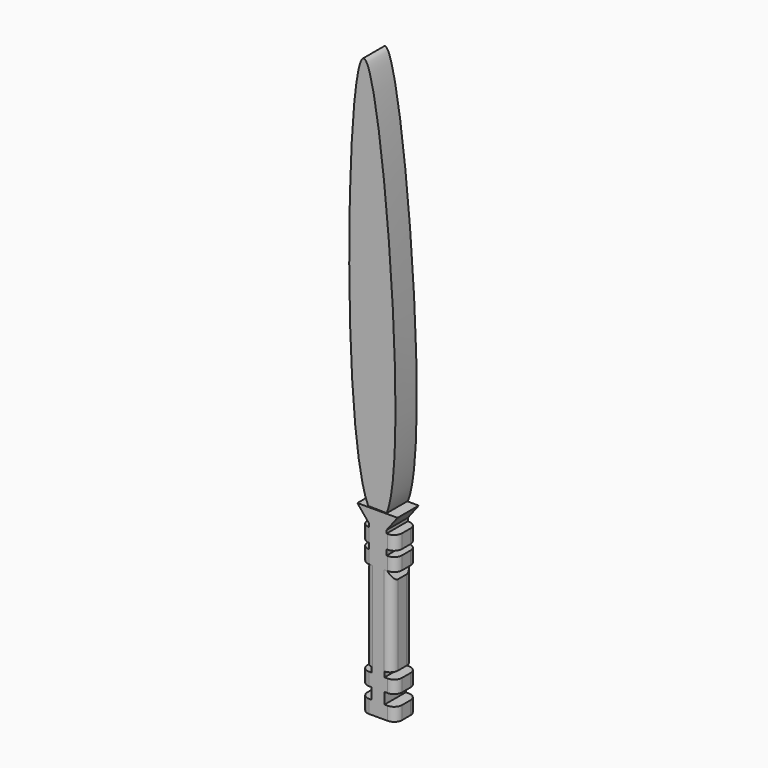
from build123d import *

# Parameters (mm, degrees)
F0_W         = 12.4557644932
F0_H         = 4.9433471202
F0_H_2       = 12.250360247
F0_W_2       = 9.9614109216
F0_W_3       = 7.6852417854
F0_H_3       = 12.623509512
F0_W_4       = 10.6767713383
F0_H_4       = 10.6608381902
F0_W_5       = 8.7539301689
F0_W_6       = 16.6547747988
F0_H_5       = 5.3106732666
F0_H_6       = 6.5328691769
F0_H_7       = 13.2375769317
F0_H_8       = 2.9359683394
F1_DEPTH     = 25.4
F2_T1_DEPTH  = 50.723509512
F2_T3_DEPTH  = 32.2875769317
F2_T5_DEPTH  = 50.350360247
F2_T7_DEPTH  = 50.8284377813
F2_T12_DEPTH = 115.0326763547
F2_T18_DEPTH = 115.0326763547
F2_T24_DEPTH = 115.0326763547
F2_T30_DEPTH = 115.0326763547
F2_T36_DEPTH = 51.3375769317
F2_T41_DEPTH = 51.3375769317
F4_DEPTH     = 25.4


# Not quite as in the source:
# - a fillet or chamfer that OpenCascade refuses, or shapes differently, is made with other operations: its cross-section is extruded or revolved along the edge and cut away or added


with BuildPart() as f1:
    # F0 (on Front) → F1 (new body)
    with BuildSketch(Plane.XZ):
        Polygon((-26.0105736841, 17.9509583747), (-26.0105736841, -58.98171798), (-19.4163457188, -58.98171798), (-6.9605812255, -58.98171798), (0, -58.98171798), (0, 17.9509583747), align=None)
        with Locations((-13.1884634722, -61.4533915401)):
            Rectangle(F0_W, F0_H)
        Polygon((-21.6925148549, 26.5870782279), (-26.0105736841, 17.9509583747), (0, 17.9509583747), (-5.0377400561, 26.5870782279), (-19.4163457188, 26.5870782279), align=None)
        with Locations((-13.1884634722, -70.0502452237)):
            Rectangle(F0_W, F0_H_2)
        with Locations((-24.3970511795, -70.0502452237)):
            Rectangle(F0_W_2, F0_H_2)
        Polygon((-21.6925148549, 39.2105877399), (-21.6925148549, 26.5870782279), (-19.4163457188, 26.5870782279), (-5.0377400561, 26.5870782279), (-5.0377400561, 39.2105877399), align=None)
        with Locations((-25.5351357476, 32.8988329839)):
            Rectangle(F0_W_3, F0_H_3)
        with Locations((-1.6221955564, -70.0502452237)):
            Rectangle(F0_W_4, F0_H_2)
        with Locations((-13.1884634722, -81.5058444423)):
            Rectangle(F0_W, F0_H_4)
        with Locations((-0.6607749717, 32.8988329839)):
            Rectangle(F0_W_5, F0_H_3)
        with Locations((-13.3651274555, 41.8659243733)):
            Rectangle(F0_W_6, F0_H_5)
        with Locations((-13.1884634722, -90.1026981259)):
            Rectangle(F0_W, F0_H_6)
        Polygon((-19.4163457188, -93.3691327143), (-19.4163457188, -86.8362635374), (-29.3777566403, -86.8362635374), (-29.3777566403, -99.5647013187), (3.7161901128, -99.5647013187), (3.7161901128, -86.8362635374), (-6.9605812255, -86.8362635374), (-6.9605812255, -93.3691327143), align=None)
        with Locations((-13.3651274555, 51.1400494725)):
            Rectangle(F0_W_6, F0_H_7)
        with Locations((-25.5351357476, 51.1400494725)):
            Rectangle(F0_W_3, F0_H_7)
        with Locations((-0.6607749717, 51.1400494725)):
            Rectangle(F0_W_5, F0_H_7)
        with Locations((-13.3651274555, 59.226822108)):
            Rectangle(F0_W_6, F0_H_8)
        Polygon((-32.9307243228, 74.4306147099), (-21.6925148549, 60.6948062778), (-5.0377400561, 60.6948062778), (5.4591065273, 74.4306147099), align=None)
    extrude(amount=F1_DEPTH)

    # F2: fillet of radius 7.62 on 20 edges, made by hand

    # F2_s2 → F2_t1 (cut)
    with BuildSketch(Plane.XY.offset(7.5370782279)):
        with BuildLine():
            ThreePointArc((3.7161901128, -17.78), (1.4843437854, -23.1681536726), (-3.9038098872, -25.4))
            Line((-3.9038098872, -25.4), (3.7161901128, -25.4))
            Line((3.7161901128, -25.4), (3.7161901128, -17.78))
        make_face()
        with BuildLine():
            ThreePointArc((3.7161901128, -7.62), (1.4843437854, -2.2318463274), (-3.9038098872, 0))
            Line((-3.9038098872, 0), (3.7161901128, 0))
            Line((3.7161901128, 0), (3.7161901128, -7.62))
        make_face()
        with BuildLine():
            ThreePointArc((-29.3777566403, -17.78), (-27.145910313, -23.1681536726), (-21.7577566403, -25.4))
            Line((-21.7577566403, -25.4), (-29.3777566403, -25.4))
            Line((-29.3777566403, -25.4), (-29.3777566403, -17.78))
        make_face()
        with BuildLine():
            ThreePointArc((-29.3777566403, -7.62), (-27.145910313, -2.2318463274), (-21.7577566403, 0))
            Line((-21.7577566403, 0), (-29.3777566403, 0))
            Line((-29.3777566403, 0), (-29.3777566403, -7.62))
        make_face()
    extrude(amount=F2_T1_DEPTH, mode=Mode.SUBTRACT)

    # F2_s4 → F2_t3 (cut)
    with BuildSketch(Plane.XY.offset(25.4712610066)):
        with BuildLine():
            ThreePointArc((-29.3777566403, -17.78), (-27.145910313, -23.1681536726), (-21.7577566403, -25.4))
            Line((-21.7577566403, -25.4), (-29.3777566403, -25.4))
            Line((-29.3777566403, -25.4), (-29.3777566403, -17.78))
        make_face()
        with BuildLine():
            ThreePointArc((-29.3777566403, -7.62), (-27.145910313, -2.2318463274), (-21.7577566403, 0))
            Line((-21.7577566403, 0), (-29.3777566403, 0))
            Line((-29.3777566403, 0), (-29.3777566403, -7.62))
        make_face()
    extrude(amount=F2_T3_DEPTH, mode=Mode.SUBTRACT)

    # F2_s6 → F2_t5 (cut)
    with BuildSketch(Plane.XY.offset(-95.2254253472)):
        with BuildLine():
            ThreePointArc((3.7161901128, -17.78), (1.4843437854, -23.1681536726), (-3.9038098872, -25.4))
            Line((-3.9038098872, -25.4), (3.7161901128, -25.4))
            Line((3.7161901128, -25.4), (3.7161901128, -17.78))
        make_face()
        with BuildLine():
            ThreePointArc((-29.3777566403, -17.78), (-27.145910313, -23.1681536726), (-21.7577566403, -25.4))
            Line((-21.7577566403, -25.4), (-29.3777566403, -25.4))
            Line((-29.3777566403, -25.4), (-29.3777566403, -17.78))
        make_face()
        with BuildLine():
            ThreePointArc((3.7161901128, -7.62), (1.4843437854, -2.2318463274), (-3.9038098872, 0))
            Line((-3.9038098872, 0), (3.7161901128, 0))
            Line((3.7161901128, 0), (3.7161901128, -7.62))
        make_face()
        with BuildLine():
            ThreePointArc((-29.3777566403, -7.62), (-27.145910313, -2.2318463274), (-21.7577566403, 0))
            Line((-21.7577566403, 0), (-29.3777566403, 0))
            Line((-29.3777566403, 0), (-29.3777566403, -7.62))
        make_face()
    extrude(amount=F2_T5_DEPTH, mode=Mode.SUBTRACT)

    # F2_s8 → F2_t7 (cut)
    with BuildSketch(Plane.XY.offset(-118.6147013187)):
        with BuildLine():
            ThreePointArc((-29.3777566403, -17.78), (-27.145910313, -23.1681536726), (-21.7577566403, -25.4))
            Line((-21.7577566403, -25.4), (-29.3777566403, -25.4))
            Line((-29.3777566403, -25.4), (-29.3777566403, -17.78))
        make_face()
        with BuildLine():
            ThreePointArc((3.7161901128, -17.78), (1.4843437854, -23.1681536726), (-3.9038098872, -25.4))
            Line((-3.9038098872, -25.4), (3.7161901128, -25.4))
            Line((3.7161901128, -25.4), (3.7161901128, -17.78))
        make_face()
        with BuildLine():
            ThreePointArc((3.7161901128, -7.62), (1.4843437854, -2.2318463274), (-3.9038098872, 0))
            Line((-3.9038098872, 0), (3.7161901128, 0))
            Line((3.7161901128, 0), (3.7161901128, -7.62))
        make_face()
        with BuildLine():
            ThreePointArc((-29.3777566403, -7.62), (-27.145910313, -2.2318463274), (-21.7577566403, 0))
            Line((-21.7577566403, 0), (-29.3777566403, 0))
            Line((-29.3777566403, 0), (-29.3777566403, -7.62))
        make_face()
    extrude(amount=F2_T7_DEPTH, mode=Mode.SUBTRACT)


with BuildPart() as f2_tool10:
    # F2_s11 → F2_t12 (new body)
    with BuildSketch(Plane.XY.offset(-78.03171798)):
        with BuildLine():
            ThreePointArc((0, -17.78), (-2.2318463274, -23.1681536726), (-7.62, -25.4))
            Line((-7.62, -25.4), (0, -25.4))
            Line((0, -25.4), (0, -17.78))
        make_face()
    extrude(amount=F2_T12_DEPTH)

    split(bisect_by=Plane.XY.offset(-63.9250651002), keep=Keep.TOP)

    split(bisect_by=Plane.XY.offset(26.5870782279), keep=Keep.BOTTOM)


with BuildPart() as f1_1:
    add(f1.part)

    # F2_t9: cut F2_tool10
    add(f2_tool10.part, mode=Mode.SUBTRACT)


with BuildPart() as f2_tool16:
    # F2_s17 → F2_t18 (new body)
    with BuildSketch(Plane.XY.offset(37.0009583747)):
        with BuildLine():
            ThreePointArc((-26.0105736841, -17.78), (-23.7787273568, -23.1681536726), (-18.3905736841, -25.4))
            Line((-18.3905736841, -25.4), (-26.0105736841, -25.4))
            Line((-26.0105736841, -25.4), (-26.0105736841, -17.78))
        make_face()
    extrude(amount=-F2_T18_DEPTH)

    split(bisect_by=Plane.XY.offset(-63.9250651002), keep=Keep.TOP)

    split(bisect_by=Plane.XY.offset(26.5870782279), keep=Keep.BOTTOM)


with BuildPart() as f1_2:
    add(f1_1.part)

    # F2_t15: cut F2_tool16
    add(f2_tool16.part, mode=Mode.SUBTRACT)


with BuildPart() as f2_tool22:
    # F2_s23 → F2_t24 (new body)
    with BuildSketch(Plane.XY.offset(37.0009583747)):
        with BuildLine():
            ThreePointArc((-26.0105736841, -7.62), (-23.7787273568, -2.2318463274), (-18.3905736841, 0))
            Line((-18.3905736841, 0), (-26.0105736841, 0))
            Line((-26.0105736841, 0), (-26.0105736841, -7.62))
        make_face()
    extrude(amount=-F2_T24_DEPTH)

    split(bisect_by=Plane.XY.offset(-63.9250651002), keep=Keep.TOP)

    split(bisect_by=Plane.XY.offset(26.5870782279), keep=Keep.BOTTOM)


with BuildPart() as f1_3:
    add(f1_2.part)

    # F2_t21: cut F2_tool22
    add(f2_tool22.part, mode=Mode.SUBTRACT)


with BuildPart() as f2_tool28:
    # F2_s29 → F2_t30 (new body)
    with BuildSketch(Plane.XY.offset(-78.03171798)):
        with BuildLine():
            ThreePointArc((0, -7.62), (-2.2318463274, -2.2318463274), (-7.62, 0))
            Line((-7.62, 0), (0, 0))
            Line((0, 0), (0, -7.62))
        make_face()
    extrude(amount=F2_T30_DEPTH)

    split(bisect_by=Plane.XY.offset(-63.9250651002), keep=Keep.TOP)

    split(bisect_by=Plane.XY.offset(26.5870782279), keep=Keep.BOTTOM)


with BuildPart() as f1_4:
    add(f1_3.part)

    # F2_t27: cut F2_tool28
    add(f2_tool28.part, mode=Mode.SUBTRACT)


with BuildPart() as f2_tool34:
    # F2_s35 → F2_t36 (new body)
    with BuildSketch(Plane.XY.offset(25.4712610066)):
        with BuildLine():
            ThreePointArc((3.7161901128, -17.78), (1.4843437854, -23.1681536726), (-3.9038098872, -25.4))
            Line((-3.9038098872, -25.4), (3.7161901128, -25.4))
            Line((3.7161901128, -25.4), (3.7161901128, -17.78))
        make_face()
    extrude(amount=F2_T36_DEPTH)

    split(bisect_by=Plane(origin=(-32.4625068275, 0, 24.8077101224), x_dir=(0, 1, 0), z_dir=(0.7945533712, 0, -0.6071943185)), keep=Keep.TOP)


with BuildPart() as f1_5:
    add(f1_4.part)

    # F2_t33: cut F2_tool34
    add(f2_tool34.part, mode=Mode.SUBTRACT)


with BuildPart() as f2_tool39:
    # F2_s40 → F2_t41 (new body)
    with BuildSketch(Plane.XY.offset(25.4712610066)):
        with BuildLine():
            ThreePointArc((3.7161901128, -7.62), (1.4843437854, -2.2318463274), (-3.9038098872, 0))
            Line((-3.9038098872, 0), (3.7161901128, 0))
            Line((3.7161901128, 0), (3.7161901128, -7.62))
        make_face()
    extrude(amount=F2_T41_DEPTH)

    split(bisect_by=Plane(origin=(-32.4625068275, 0, 24.8077101224), x_dir=(0, 1, 0), z_dir=(0.7945533712, 0, -0.6071943185)), keep=Keep.TOP)


with BuildPart() as f1_6:
    add(f1_5.part)

    # F2_t38: cut F2_tool39
    add(f2_tool39.part, mode=Mode.SUBTRACT)


with BuildPart() as f4:
    # F3 (on Front) → F4 (new body)
    with BuildSketch(Plane.XZ):
        with BuildLine():
            add(Edge.make_bspline(
                [(-4.8297718167, 75.0046595931), (17.4862886619, 131.4259865322), (-37.8070554952, 769.294306067), (-48.8232825035, 132.7576780254), (-22.5946810097, 75.3747597337)],
                knots=[0.0980571238, 0.0980571238, 0.0980571238, 0.0980571238, 0.5493244895, 1, 1, 1, 1], degree=3))
            add(Edge.make_bspline(
                [(-4.8297718167, 75.0046595931), (-10.7514082144, 75.1280263066), (-16.673044612, 75.2513930202), (-22.5946810097, 75.3747597337)],
                knots=[0, 0, 0, 0, 17.7687639623, 17.7687639623, 17.7687639623, 17.7687639623], degree=3))
        make_face()
    extrude(amount=F4_DEPTH)


solid = Compound([f1_6.part, f4.part])
